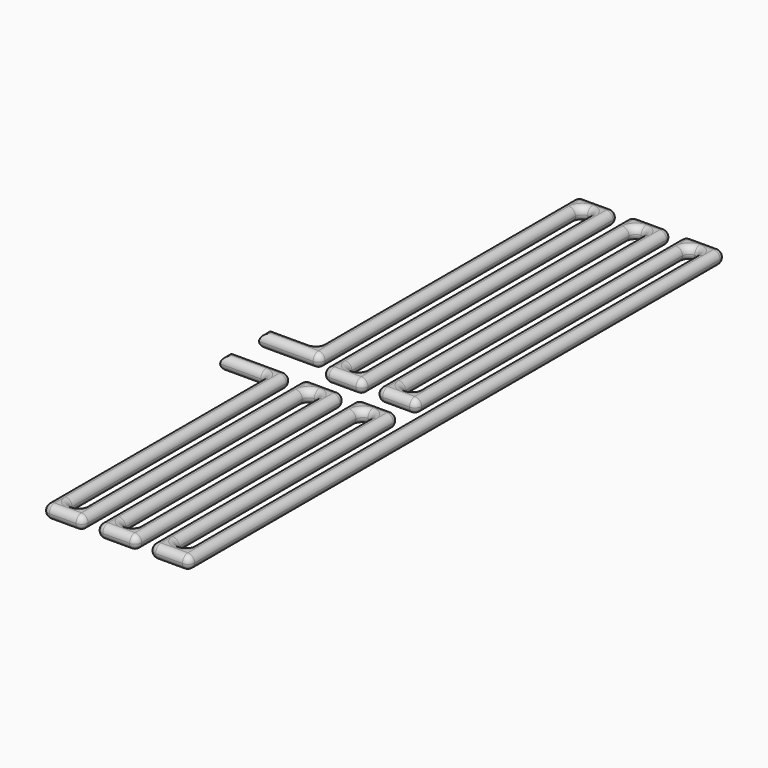
from build123d import *

# Parameters (mm, degrees)
F1_DEPTH = 5
F2_R     = 2.49999


# Not quite as in the source:
# - a fillet or chamfer is up to 0.001 mm smaller than in the source, because OpenCascade refuses the exact size


with BuildPart() as f1:
    # F0 (on Top) → F1 (new body)
    with BuildSketch(Plane.XY):
        with BuildLine():
            Line((0, 5), (0, 0))
            Line((0, 0), (17.6796003883, 0))
            Line((17.6796003883, 0), (20.1796003883, 0))
            ThreePointArc((20.1796003883, 0), (21.9473673413, 0.732233047), (22.6796003883, 2.5))
            Line((22.6796003883, 2.5), (22.6796003883, 119.3484082763))
            ThreePointArc((22.6796003883, 119.3484082763), (23.4118334353, 121.1161752293), (25.1796003883, 121.8484082763))
            ThreePointArc((25.1796003883, 121.8484082763), (26.9473673413, 121.1161752293), (27.6796003883, 119.3484082763))
            Line((27.6796003883, 119.3484082763), (27.6796003883, 0))
            Line((27.6796003883, 0), (27.6796003883, -2.5))
            ThreePointArc((27.6796003883, -2.5), (28.4118334353, -4.267766953), (30.1796003883, -5))
            Line((30.1796003883, -5), (40.1796003883, -5))
            ThreePointArc((40.1796003883, -5), (41.9473673413, -4.267766953), (42.6796003883, -2.5))
            Line((42.6796003883, -2.5), (42.6796003883, 0))
            Line((42.6796003883, 0), (42.6796003883, 119.3484082763))
            ThreePointArc((42.6796003883, 119.3484082763), (43.4118334353, 121.1161752293), (45.1796003883, 121.8484082763))
            ThreePointArc((45.1796003883, 121.8484082763), (46.9473673413, 121.1161752293), (47.6796003883, 119.3484082763))
            Line((47.6796003883, 119.3484082763), (47.6796003883, 0))
            Line((47.6796003883, 0), (47.6796003883, -2.5))
            ThreePointArc((47.6796003883, -2.5), (48.4118334353, -4.267766953), (50.1796003883, -5))
            Line((50.1796003883, -5), (60.1796003883, -5))
            ThreePointArc((60.1796003883, -5), (61.9473673413, -4.267766953), (62.6796003883, -2.5))
            Line((62.6796003883, -2.5), (62.6796003883, 0))
            Line((62.6796003883, 0), (62.6796003883, 119.3484082763))
            ThreePointArc((62.6796003883, 119.3484082763), (63.4118334353, 121.1161752293), (65.1796003883, 121.8484082763))
            ThreePointArc((65.1796003883, 121.8484082763), (66.9473673413, 121.1161752293), (67.6796003883, 119.3484082763))
            Line((67.6796003883, 119.3484082763), (67.6796003883, -115.6515917237))
            ThreePointArc((67.6796003883, -115.6515917237), (66.9473673413, -117.4193586767), (65.1796003883, -118.1515917237))
            ThreePointArc((65.1796003883, -118.1515917237), (63.4118334353, -117.4193586767), (62.6796003883, -115.6515917237))
            Line((62.6796003883, -115.6515917237), (62.6796003883, -18.1515917237))
            Line((62.6796003883, -18.1515917237), (62.6796003883, -15.6515917237))
            ThreePointArc((62.6796003883, -15.6515917237), (61.9473673413, -13.8838247707), (60.1796003883, -13.1515917237))
            Line((60.1796003883, -13.1515917237), (50.1796003883, -13.1515917237))
            ThreePointArc((50.1796003883, -13.1515917237), (48.4118334353, -13.8838247707), (47.6796003883, -15.6515917237))
            Line((47.6796003883, -15.6515917237), (47.6796003883, -18.1515917237))
            Line((47.6796003883, -18.1515917237), (47.6796003883, -115.6515917237))
            ThreePointArc((47.6796003883, -115.6515917237), (46.9473673413, -117.4193586767), (45.1796003883, -118.1515917237))
            ThreePointArc((45.1796003883, -118.1515917237), (43.4118334353, -117.4193586767), (42.6796003883, -115.6515917237))
            Line((42.6796003883, -115.6515917237), (42.6796003883, -18.1515917237))
            Line((42.6796003883, -18.1515917237), (42.6796003883, -15.6515917237))
            ThreePointArc((42.6796003883, -15.6515917237), (41.9473673413, -13.8838247707), (40.1796003883, -13.1515917237))
            Line((40.1796003883, -13.1515917237), (30.1796003883, -13.1515917237))
            ThreePointArc((30.1796003883, -13.1515917237), (28.4118334353, -13.8838247707), (27.6796003883, -15.6515917237))
            Line((27.6796003883, -15.6515917237), (27.6796003883, -18.1515917237))
            Line((27.6796003883, -18.1515917237), (27.6796003883, -115.6515917237))
            ThreePointArc((27.6796003883, -115.6515917237), (26.9473673413, -117.4193586767), (25.1796003883, -118.1515917237))
            ThreePointArc((25.1796003883, -118.1515917237), (23.4118334353, -117.4193586767), (22.6796003883, -115.6515917237))
            Line((22.6796003883, -115.6515917237), (22.6796003883, -18.1515917237))
            Line((22.6796003883, -18.1515917237), (22.6796003883, -15.6515917237))
            ThreePointArc((22.6796003883, -15.6515917237), (21.9473673413, -13.8838247707), (20.1796003883, -13.1515917237))
            Line((20.1796003883, -13.1515917237), (0, -13.1515917237))
            Line((0, -13.1515917237), (0, -18.1515917237))
            Line((0, -18.1515917237), (15.1796003883, -18.1515917237))
            ThreePointArc((15.1796003883, -18.1515917237), (16.9473673413, -18.8838247707), (17.6796003883, -20.6515917237))
            Line((17.6796003883, -20.6515917237), (17.6796003883, -118.1515917237))
            Line((17.6796003883, -118.1515917237), (17.6796003883, -120.6515917237))
            ThreePointArc((17.6796003883, -120.6515917237), (18.4118334353, -122.4193586767), (20.1796003883, -123.1515917237))
            Line((20.1796003883, -123.1515917237), (30.1796003883, -123.1515917237))
            ThreePointArc((30.1796003883, -123.1515917237), (31.9473673413, -122.4193586767), (32.6796003883, -120.6515917237))
            Line((32.6796003883, -120.6515917237), (32.6796003883, -118.1515917237))
            Line((32.6796003883, -118.1515917237), (32.6796003883, -20.6515917237))
            ThreePointArc((32.6796003883, -20.6515917237), (33.4118334353, -18.8838247707), (35.1796003883, -18.1515917237))
            ThreePointArc((35.1796003883, -18.1515917237), (36.9473673413, -18.8838247707), (37.6796003883, -20.6515917237))
            Line((37.6796003883, -20.6515917237), (37.6796003883, -118.1515917237))
            Line((37.6796003883, -118.1515917237), (37.6796003883, -120.6515917237))
            ThreePointArc((37.6796003883, -120.6515917237), (38.4118334353, -122.4193586767), (40.1796003883, -123.1515917237))
            Line((40.1796003883, -123.1515917237), (50.1796003883, -123.1515917237))
            ThreePointArc((50.1796003883, -123.1515917237), (51.9473673413, -122.4193586767), (52.6796003883, -120.6515917237))
            Line((52.6796003883, -120.6515917237), (52.6796003883, -118.1515917237))
            Line((52.6796003883, -118.1515917237), (52.6796003883, -20.6515917237))
            ThreePointArc((52.6796003883, -20.6515917237), (53.4118334353, -18.8838247707), (55.1796003883, -18.1515917237))
            ThreePointArc((55.1796003883, -18.1515917237), (56.9473673413, -18.8838247707), (57.6796003883, -20.6515917237))
            Line((57.6796003883, -20.6515917237), (57.6796003883, -118.1515917237))
            Line((57.6796003883, -118.1515917237), (57.6796003883, -120.9787243429))
            ThreePointArc((57.6796003883, -120.9787243429), (58.4118334353, -122.7464912959), (60.1796003883, -123.4787243429))
            Line((60.1796003883, -123.4787243429), (70.1796003883, -123.4787243429))
            ThreePointArc((70.1796003883, -123.4787243429), (71.9473673413, -122.7464912959), (72.6796003883, -120.9787243429))
            Line((72.6796003883, -120.9787243429), (72.6796003883, -118.1515917237))
            Line((72.6796003883, -118.1515917237), (72.6796003883, 121.8484082763))
            Line((72.6796003883, 121.8484082763), (72.6796003883, 124.3484082763))
            ThreePointArc((72.6796003883, 124.3484082763), (71.9473673413, 126.1161752293), (70.1796003883, 126.8484082763))
            Line((70.1796003883, 126.8484082763), (60.1796003883, 126.8484082763))
            ThreePointArc((60.1796003883, 126.8484082763), (58.4118334353, 126.1161752293), (57.6796003883, 124.3484082763))
            Line((57.6796003883, 124.3484082763), (57.6796003883, 121.8484082763))
            Line((57.6796003883, 121.8484082763), (57.6796003883, 2.5))
            ThreePointArc((57.6796003883, 2.5), (56.9473673413, 0.732233047), (55.1796003883, 0))
            ThreePointArc((55.1796003883, 0), (53.4118334353, 0.732233047), (52.6796003883, 2.5))
            Line((52.6796003883, 2.5), (52.6796003883, 121.8484082763))
            Line((52.6796003883, 121.8484082763), (52.6796003883, 124.3484082763))
            ThreePointArc((52.6796003883, 124.3484082763), (51.9473673413, 126.1161752293), (50.1796003883, 126.8484082763))
            Line((50.1796003883, 126.8484082763), (40.1796003883, 126.8484082763))
            ThreePointArc((40.1796003883, 126.8484082763), (38.4118334353, 126.1161752293), (37.6796003883, 124.3484082763))
            Line((37.6796003883, 124.3484082763), (37.6796003883, 121.8484082763))
            Line((37.6796003883, 121.8484082763), (37.6796003883, 2.5))
            ThreePointArc((37.6796003883, 2.5), (36.9473673413, 0.732233047), (35.1796003883, 0))
            ThreePointArc((35.1796003883, 0), (33.4118334353, 0.732233047), (32.6796003883, 2.5))
            Line((32.6796003883, 2.5), (32.6796003883, 121.8484082763))
            Line((32.6796003883, 121.8484082763), (32.6796003883, 124.3484082763))
            ThreePointArc((32.6796003883, 124.3484082763), (31.9473673413, 126.1161752293), (30.1796003883, 126.8484082763))
            Line((30.1796003883, 126.8484082763), (20.1796003883, 126.8484082763))
            ThreePointArc((20.1796003883, 126.8484082763), (18.4118334353, 126.1161752293), (17.6796003883, 124.3484082763))
            Line((17.6796003883, 124.3484082763), (17.6796003883, 121.8484082763))
            Line((17.6796003883, 121.8484082763), (17.6796003883, 7.5))
            ThreePointArc((17.6796003883, 7.5), (16.9473673413, 5.732233047), (15.1796003883, 5))
            Line((15.1796003883, 5), (0, 5))
        make_face()
    extrude(amount=F1_DEPTH)

    # F2 (radius 2.5 in the source; OpenCascade refuses exactly that, so slightly less here)
    f2_edges = [f1.edges().sort_by_distance(p)[0] for p in [
        (25.1796, 126.848408, 5),
        (18.411833, 126.116175, 5),
        (17.6796, 65.924204, 5),
        (16.947367, 5.732233, 5),
        (7.5898, 5, 5),
        (0, 2.5, 5),
        (10.0898, 0, 5),
        (21.947367, 0.732233, 5),
        (22.6796, 60.924204, 5),
        (25.1796, 121.848408, 5),
        (27.6796, 58.424204, 5),
        (28.411833, -4.267767, 5),
        (35.1796, -5, 5),
        (41.947367, -4.267767, 5),
        (42.6796, 58.424204, 5),
        (45.1796, 121.848408, 5),
        (47.6796, 58.424204, 5),
        (48.411833, -4.267767, 5),
        (55.1796, -5, 5),
        (61.947367, -4.267767, 5),
        (62.6796, 58.424204, 5),
        (65.1796, 121.848408, 5),
        (67.6796, 1.848408, 5),
        (65.1796, -118.151592, 5),
        (62.6796, -65.651592, 5),
        (61.947367, -13.883825, 5),
        (55.1796, -13.151592, 5),
        (48.411833, -13.883825, 5),
        (47.6796, -65.651592, 5),
        (45.1796, -118.151592, 5),
        (42.6796, -65.651592, 5),
        (41.947367, -13.883825, 5),
        (35.1796, -13.151592, 5),
        (28.411833, -13.883825, 5),
        (27.6796, -65.651592, 5),
        (25.1796, -118.151592, 5),
        (22.6796, -65.651592, 5),
        (21.947367, -13.883825, 5),
        (10.0898, -13.151592, 5),
        (0, -15.651592, 5),
        (7.5898, -18.151592, 5),
        (16.947367, -18.883825, 5),
        (17.6796, -70.651592, 5),
        (18.411833, -122.419359, 5),
        (25.1796, -123.151592, 5),
        (31.947367, -122.419359, 5),
        (32.6796, -70.651592, 5),
        (35.1796, -18.151592, 5),
        (37.6796, -70.651592, 5),
        (38.411833, -122.419359, 5),
        (45.1796, -123.151592, 5),
        (51.947367, -122.419359, 5),
        (52.6796, -70.651592, 5),
        (55.1796, -18.151592, 5),
        (57.6796, -70.815158, 5),
        (58.411833, -122.746491, 5),
        (65.1796, -123.478724, 5),
        (71.947367, -122.746491, 5),
        (72.6796, 1.684842, 5),
        (71.947367, 126.116175, 5),
        (65.1796, 126.848408, 5),
        (58.411833, 126.116175, 5),
        (57.6796, 63.424204, 5),
        (55.1796, 0, 5),
        (52.6796, 63.424204, 5),
        (51.947367, 126.116175, 5),
        (45.1796, 126.848408, 5),
        (38.411833, 126.116175, 5),
        (37.6796, 63.424204, 5),
        (35.1796, 0, 5),
        (32.6796, 63.424204, 5),
        (31.947367, 126.116175, 5),
        (25.1796, 126.848408, 0),
        (18.411833, 126.116175, 0),
        (17.6796, 65.924204, 0),
        (16.947367, 5.732233, 0),
        (7.5898, 5, 0),
        (0, 2.5, 0),
        (10.0898, 0, 0),
        (21.947367, 0.732233, 0),
        (22.6796, 60.924204, 0),
        (25.1796, 121.848408, 0),
        (27.6796, 58.424204, 0),
        (28.411833, -4.267767, 0),
        (35.1796, -5, 0),
        (41.947367, -4.267767, 0),
        (42.6796, 58.424204, 0),
        (45.1796, 121.848408, 0),
        (47.6796, 58.424204, 0),
        (48.411833, -4.267767, 0),
        (55.1796, -5, 0),
        (61.947367, -4.267767, 0),
        (62.6796, 58.424204, 0),
        (65.1796, 121.848408, 0),
        (67.6796, 1.848408, 0),
        (65.1796, -118.151592, 0),
        (62.6796, -65.651592, 0),
        (61.947367, -13.883825, 0),
        (55.1796, -13.151592, 0),
        (48.411833, -13.883825, 0),
        (47.6796, -65.651592, 0),
        (45.1796, -118.151592, 0),
        (42.6796, -65.651592, 0),
        (41.947367, -13.883825, 0),
        (35.1796, -13.151592, 0),
        (28.411833, -13.883825, 0),
        (27.6796, -65.651592, 0),
        (25.1796, -118.151592, 0),
        (22.6796, -65.651592, 0),
        (21.947367, -13.883825, 0),
        (10.0898, -13.151592, 0),
        (0, -15.651592, 0),
        (7.5898, -18.151592, 0),
        (16.947367, -18.883825, 0),
        (17.6796, -70.651592, 0),
        (18.411833, -122.419359, 0),
        (25.1796, -123.151592, 0),
        (31.947367, -122.419359, 0),
        (32.6796, -70.651592, 0),
        (35.1796, -18.151592, 0),
        (37.6796, -70.651592, 0),
        (38.411833, -122.419359, 0),
        (45.1796, -123.151592, 0),
        (51.947367, -122.419359, 0),
        (52.6796, -70.651592, 0),
        (55.1796, -18.151592, 0),
        (57.6796, -70.815158, 0),
        (58.411833, -122.746491, 0),
        (65.1796, -123.478724, 0),
        (71.947367, -122.746491, 0),
        (72.6796, 1.684842, 0),
        (71.947367, 126.116175, 0),
        (65.1796, 126.848408, 0),
        (58.411833, 126.116175, 0),
        (57.6796, 63.424204, 0),
        (55.1796, 0, 0),
        (52.6796, 63.424204, 0),
        (51.947367, 126.116175, 0),
        (45.1796, 126.848408, 0),
        (38.411833, 126.116175, 0),
        (37.6796, 63.424204, 0),
        (35.1796, 0, 0),
        (32.6796, 63.424204, 0),
        (31.947367, 126.116175, 0),
    ]]
    fillet(f2_edges, radius=F2_R)


solid = f1.part
